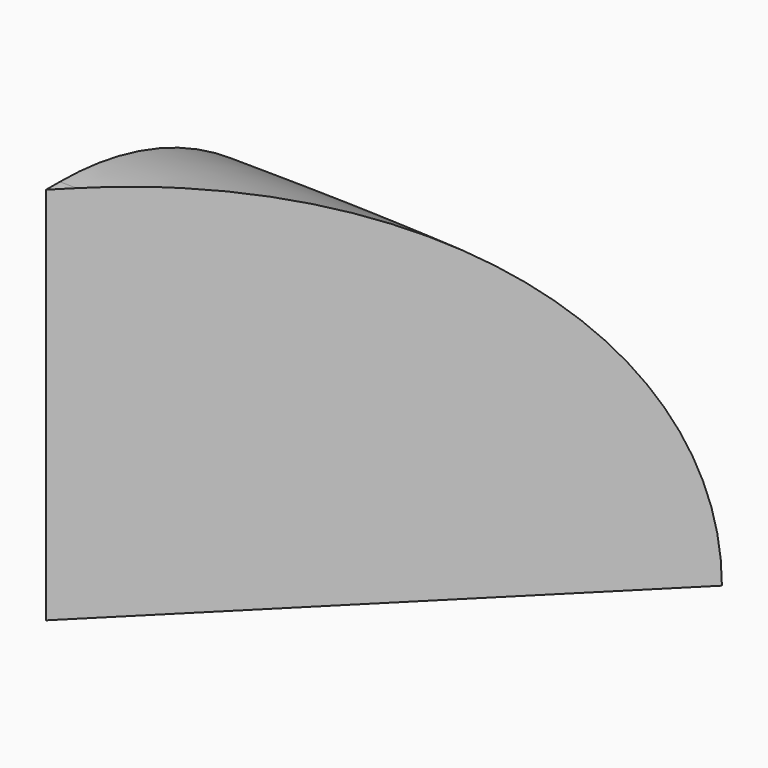
from build123d import *

# Parameters (mm, degrees)
F2_DEPTH = 25.4
F3_R     = 25.39999


# Not quite as in the source:
# - a fillet or chamfer is up to 0.001 mm smaller than in the source, because OpenCascade refuses the exact size


with BuildPart() as f2:
    # F1 (on face) → F2 (new body)
    with BuildSketch(Plane.XY):
        with BuildLine():
            ThreePointArc((25.1559020156, 227.2116647397), (12.5970917379, 228.2526522951), (0, 228.6))
            Line((0, 228.6), (0, 202.0557627241))
            Line((0, 202.0557627241), (25.1559020156, 227.2116647397))
        make_face()
    extrude(amount=F2_DEPTH)

    # F3 (radius 25.4 in the source; OpenCascade refuses exactly that, so slightly less here)
    f3_edges = [f2.edges().sort_by_distance(p)[0] for p in [
        (12.597092, 228.252652, 25.4),
    ]]
    fillet(f3_edges, radius=F3_R)


solid = f2.part
